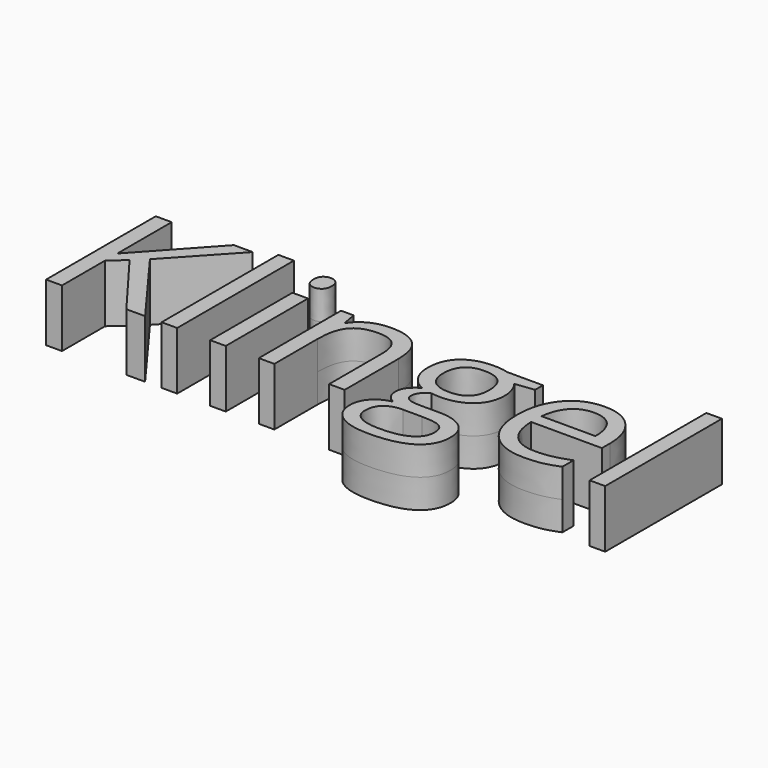
from build123d import *

# Parameters (mm, degrees)
F0_TEXT_SIZE  = 168.7764293618
F1_DEPTH      = 25.4
F1_DEPTH_BACK = 25.4


# Not quite as in the source:
# - Text() gives the source's letters only with a copy of the font that has no kerning and outlines rounded to 1/6400 em; it was checked with that copy


with BuildPart() as f1:
    # F0 (on Top) → F1 (new body, two sides)
    with BuildSketch(Plane.XY) as f1_sk:
        with Locations((-48.9040911198, -9.8374634981)):
            Text('Klingel', F0_TEXT_SIZE, font='Open Sans', text_align=(TextAlign.LEFT, TextAlign.BOTTOM))
    extrude(amount=-F1_DEPTH)
    extrude(f1_sk.sketch, amount=F1_DEPTH_BACK)


solid = f1.part
